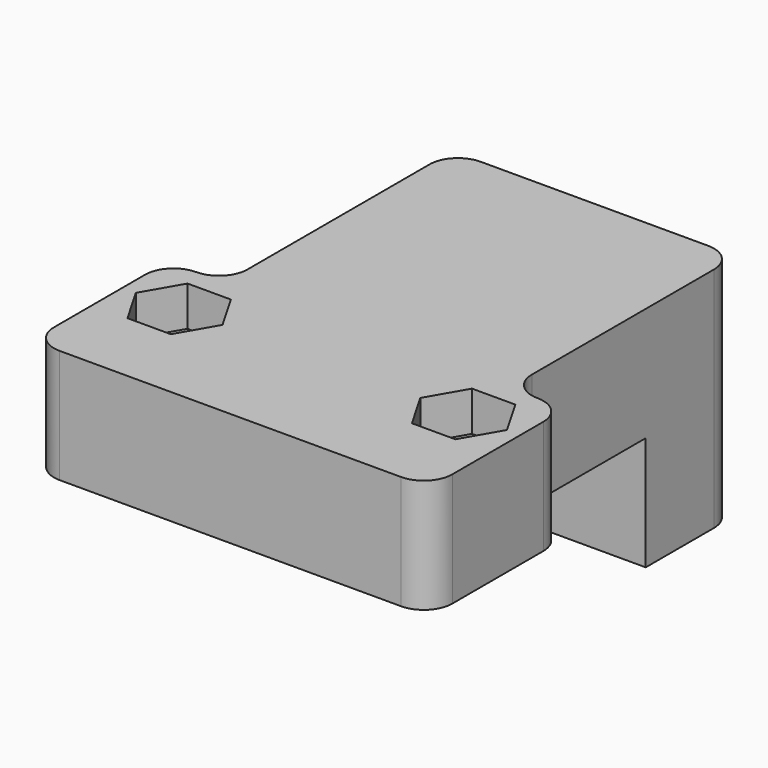
from build123d import *

# Parameters (mm, degrees)
F1_DEPTH  = 20
F3_DEPTH  = 7
F4_R      = 4
F5_DEPTH  = 13.001
F6_R      = 4
F7_DEPTH  = 20.001
F8_W      = 50
F8_H      = 20
F9_DEPTH  = 20
F10_W     = 25
F10_H     = 45
F11_DEPTH = 10
F12_R     = 4.99999


# Not quite as in the source:
# - a fillet or chamfer is up to 0.001 mm smaller than in the source, because OpenCascade refuses the exact size


with BuildPart() as f1:
    # F0 (on Top) → F1 (new body)
    with BuildSketch(Plane.XY):
        Polygon((0, 30), (0, 0), (70, 0), (70, 30), (60, 30), (60, 80), (10, 80), (10, 30), align=None)
    extrude(amount=F1_DEPTH)

    # F2 (on face) → F3 (cut)
    with BuildSketch(Plane.XY.offset(20)):
        Polygon((63.8105117767, 13.4), (67.6210235533, 20), (63.8105117767, 26.6), (56.1894882233, 26.6), (52.3789764467, 20), (56.1894882233, 13.4), align=None)
        Polygon((17.6210235533, 20), (13.8105117767, 26.6), (6.1894882233, 26.6), (2.3789764467, 20), (6.1894882233, 13.4), (13.8105117767, 13.4), align=None)
    extrude(amount=-F3_DEPTH, mode=Mode.SUBTRACT)

    # F4 (on face) → F5 (cut, through all)
    with BuildSketch(Plane.XY.offset(13)):
        with Locations((10, 20)):
            Circle(F4_R)
    extrude(amount=-F5_DEPTH, mode=Mode.SUBTRACT)

    # F6 (on face) → F7 (cut, through all)
    with BuildSketch(Plane.XY.offset(20)):
        with Locations((60, 20)):
            Circle(F6_R)
    extrude(amount=-F7_DEPTH, mode=Mode.SUBTRACT)

    # F8 (on face) → F9 (join)
    with BuildSketch(Plane(origin=(0, 0, 0), x_dir=(1, 0, 0), z_dir=(0, 0, -1))):
        with Locations((35, -70)):
            Rectangle(F8_W, F8_H)
    extrude(amount=F9_DEPTH)

    # F10 (on face) → F11 (cut)
    with BuildSketch(Plane(origin=(0, 0, 0), x_dir=(1, 0, 0), z_dir=(0, 0, -1))):
        with Locations((35, -37.5)):
            Rectangle(F10_W, F10_H)
    extrude(amount=-F11_DEPTH, mode=Mode.SUBTRACT)

    # F12 (radius 5 in the source; OpenCascade refuses exactly that, so slightly less here)
    f12_edges = [f1.edges().sort_by_distance(p)[0] for p in [
        (10, 80, 0),
        (10, 30, 10),
        (60, 30, 10),
        (70, 30, 10),
        (70, 0, 10),
        (0, 0, 10),
        (0, 30, 10),
        (60, 80, 0),
    ]]
    fillet(f12_edges, radius=F12_R)


solid = f1.part
